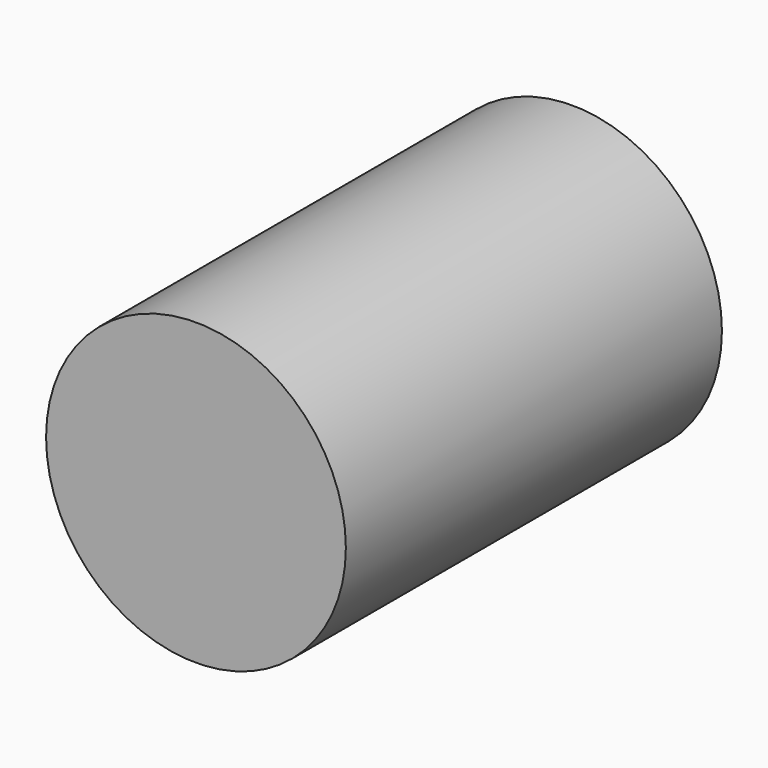
from build123d import *

# Parameters (mm, degrees)
F0_R     = 45.3527731197
F0_R_2   = 11.0004628077
F1_DEPTH = 71.12


# Not quite as in the source:
# - the program builds the solid bodies; features that only make, move or delete a surface that nothing else refers to are left out


with BuildPart() as f1:
    # F0 (on Front) → F1 (new body, symmetric)
    with BuildSketch(Plane.XZ):
        with Locations((-11.0004628077, 0)):
            Circle(F0_R)
        with Locations((-11.0004628077, 0)):
            Circle(F0_R_2, mode=Mode.SUBTRACT)
        with Locations((-11.0004628077, 0)):
            Circle(F0_R_2)
    extrude(amount=F1_DEPTH, both=True)


solid = f1.part
